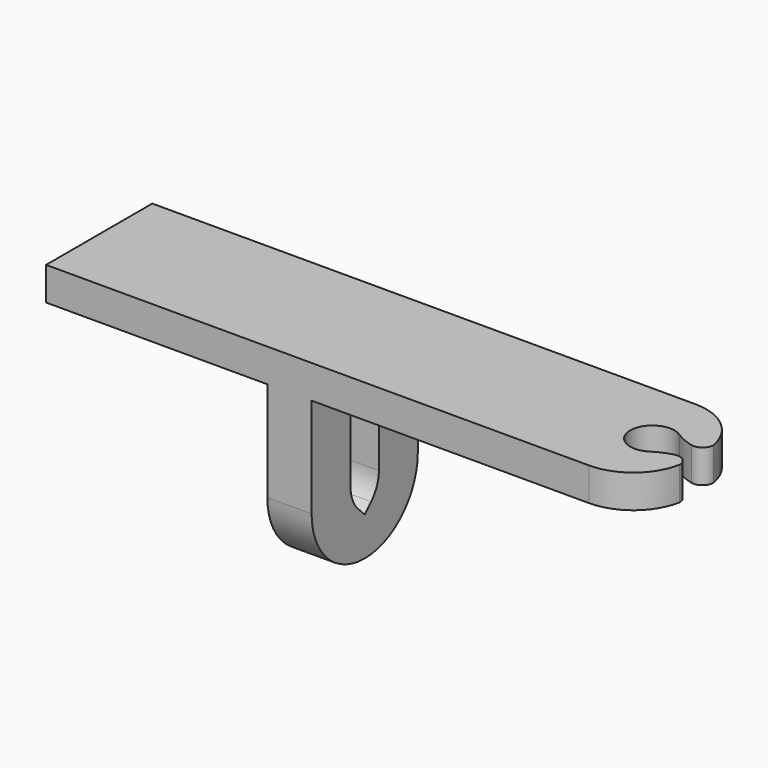
from build123d import *

# Parameters (mm, degrees)
F1_DEPTH    = 6
F3_DEPTH    = 18.001
F4_R        = 1
F5_T1_DEPTH = 27.5742386794
F7_DEPTH    = 24.001
F8_R        = 3
F9_R        = 5.99999


# Not quite as in the source:
# - a fillet or chamfer that OpenCascade refuses, or shapes differently, is made with other operations: its cross-section is extruded or revolved along the edge and cut away or added
# - a fillet or chamfer is up to 0.001 mm smaller than in the source, because OpenCascade refuses the exact size


with BuildPart() as f1:
    # F0 (on Front) → F1 (new body, symmetric)
    with BuildSketch(Plane.XZ):
        Polygon((0, -15), (0, 0), (30, 0), (30, 3), (-24, 3), (-24, 0), (-4, 0), (-4, -15), align=None)
    extrude(amount=F1_DEPTH, both=True)

    # F2 (on face) → F3 (cut, through all)
    with BuildSketch(Plane.XY.offset(3)):
        with BuildLine():
            ThreePointArc((30, 0.8), (28.4866344694, 1.0221148978), (27.1009174312, 1.6697247706))
            ThreePointArc((27.1009174312, 1.6697247706), (24, 0), (27.1009174312, -1.6697247706))
            ThreePointArc((27.1009174312, -1.6697247706), (28.4866344694, -1.0221148978), (30, -0.8))
            Line((30, -0.8), (30, 0.8))
        make_face()
    extrude(amount=-F3_DEPTH, mode=Mode.SUBTRACT)

    # F4
    f4_edges = [f1.edges().sort_by_distance(p)[0] for p in [
        (30, 0.8, 1.5),
        (30, -0.8, 1.5),
    ]]
    fillet(f4_edges, radius=F4_R)

    # F5: fillet of radius 5 on 2 edges, made by hand

    # F5_s2 → F5_t1 (cut)
    with BuildSketch(Plane.XY.offset(-12.2871193397)):
        with BuildLine():
            ThreePointArc((25.0851522641, 6), (28.2793491095, 4.8467007309), (30, 1.9188426053))
            Line((30, 1.9188426053), (30.0982969547, 1.9372194574))
            ThreePointArc((30.0982969547, 1.9372194574), (30.1, 3.9594213026), (30.1, 6))
            Line((30.1, 6), (30, 6.1))
            Line((30, 6.1), (25.0851522641, 6.1))
            Line((25.0851522641, 6.1), (25.0851522641, 6))
        make_face()
        with BuildLine():
            ThreePointArc((30, -1.9188426053), (28.2793491095, -4.8467007309), (25.0851522641, -6))
            Line((25.0851522641, -6), (25.0851522641, -6.1))
            Line((25.0851522641, -6.1), (30, -6.1))
            Line((30, -6.1), (30.1, -6))
            ThreePointArc((30.1, -6), (30.1, -3.9594213026), (30.0982969547, -1.9372194574))
            Line((30.0982969547, -1.9372194574), (30, -1.9188426053))
        make_face()
    extrude(amount=F5_T1_DEPTH, mode=Mode.SUBTRACT)

    # F6 (on face) → F7 (cut, through all)
    with BuildSketch(Plane.YZ):
        with BuildLine():
            Line((0.1, -1), (-0.1, -1))
            ThreePointArc((-0.1, -1), (-1.1606601718, -1.4393398282), (-1.6, -2.5))
            Line((-1.6, -2.5), (-1.6, -9.9))
            Line((-1.6, -9.9), (0, -11.5))
            Line((0, -11.5), (1.6, -9.9))
            Line((1.6, -9.9), (1.6, -2.5))
            ThreePointArc((1.6, -2.5), (1.1606601718, -1.4393398282), (0.1, -1))
        make_face()
    extrude(amount=-F7_DEPTH, mode=Mode.SUBTRACT)

    # F8
    f8_edges = [f1.edges().sort_by_distance(p)[0] for p in [
        (-2, -1.6, -9.9),
        (-2, 1.6, -9.9),
    ]]
    fillet(f8_edges, radius=F8_R)

    # F9 (radius 6 in the source; OpenCascade refuses exactly that, so slightly less here)
    f9_edges = [f1.edges().sort_by_distance(p)[0] for p in [
        (-2, -6, -15),
        (-2, 6, -15),
    ]]
    fillet(f9_edges, radius=F9_R)


solid = f1.part
